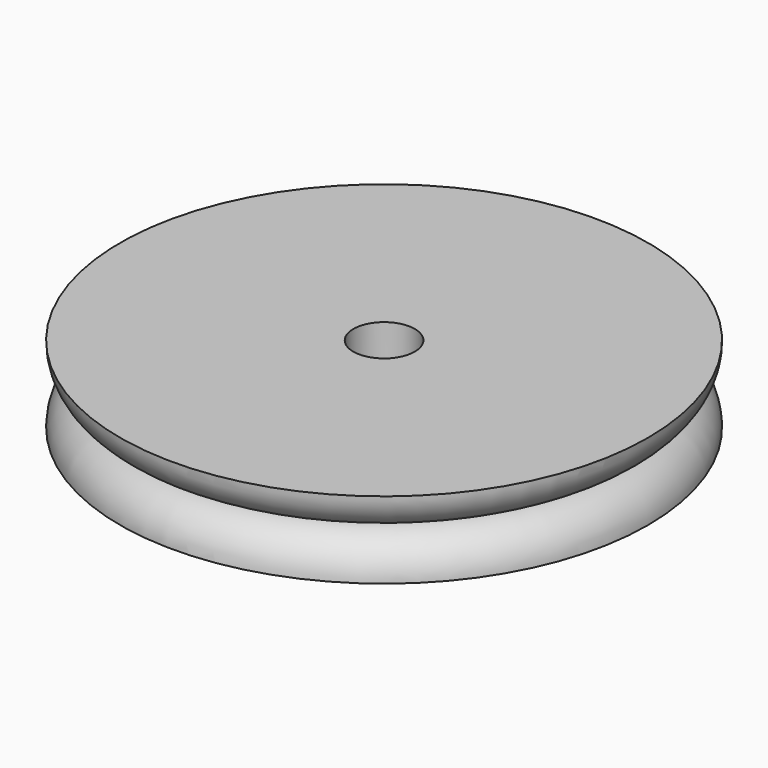
from build123d import *

# Parameters (mm, degrees)
F0_R     = 51.5
F1_DEPTH = 7.5
F2_R     = 7.49999
F3_R     = 51.5
F3_R_2   = 44.00001
F4_DEPTH = 7.5
F5_R     = 7.4999
F6_R     = 6
F7_DEPTH = 25


# Not quite as in the source:
# - a fillet or chamfer is up to 0.001 mm smaller than in the source, because OpenCascade refuses the exact size


with BuildPart() as f1:
    # F0 (on Top) → F1 (new body)
    with BuildSketch(Plane.XY):
        Circle(F0_R)
    extrude(amount=F1_DEPTH)

    # F2 (radius 7.5 in the source; OpenCascade refuses exactly that, so slightly less here)
    f2_edges = [f1.edges().sort_by_distance(p)[0] for p in [
        (-51.5, 0, 7.5),
    ]]
    fillet(f2_edges, radius=F2_R)

    # F3 (on face) → F4 (join)
    with BuildSketch(Plane.XY.offset(7.5)):
        Circle(F3_R)
        Circle(F3_R_2, mode=Mode.SUBTRACT)
        Circle(F3_R_2)
    extrude(amount=F4_DEPTH)

    # F5 (radius 7.5 in the source; OpenCascade refuses exactly that, so slightly less here)
    f5_edges = [f1.edges().sort_by_distance(p)[0] for p in [
        (-51.5, 0, 7.5),
    ]]
    fillet(f5_edges, radius=F5_R)

    # F6 (on face) → F7 (cut)
    with BuildSketch(Plane.XY.offset(15)):
        Circle(F6_R)
    extrude(amount=-F7_DEPTH, mode=Mode.SUBTRACT)


solid = f1.part
